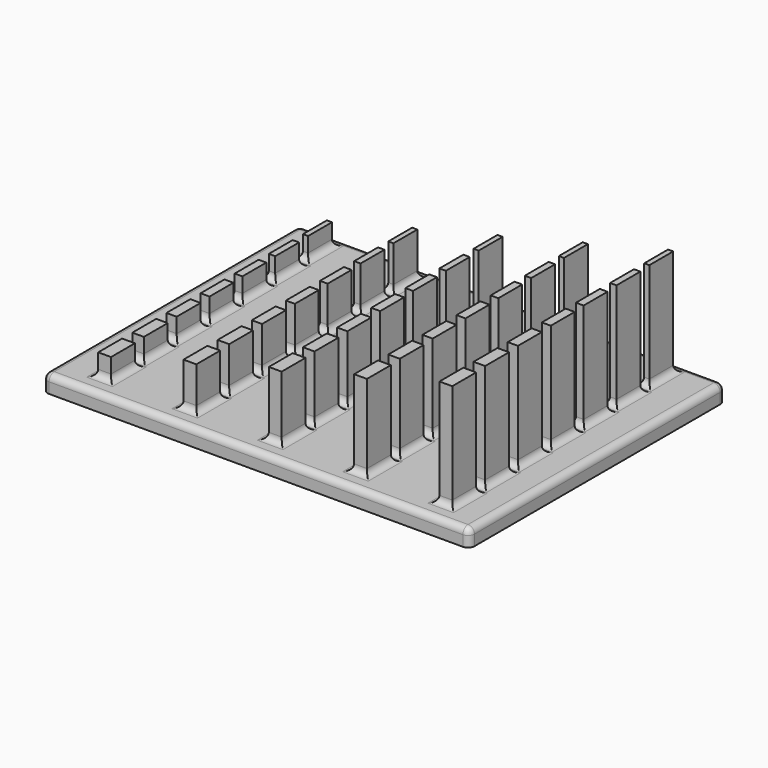
from build123d import *

# Parameters (mm, degrees)
F0_W          = 100
F0_H          = 75
F1_DEPTH      = 4
F2_W          = 2.4
F2_H          = 7
F2_W_2        = 3
F2_W_3        = 1.8
F2_W_4        = 1.2
F2_W_5        = 1.5
F2_W_6        = 2.7
F2_W_7        = 2.1
F3_DEPTH      = 5
F4_DEPTH      = 10
F5_DEPTH      = 15
F6_DEPTH      = 20
F7_DEPTH      = 25
F8_R          = 1.49999
F9_T1_DEPTH   = 7.75
F9_T4_ANGLE   = 90
F9_T6_ANGLE   = 90
F9_T8_ANGLE   = 90
F9_T10_ANGLE  = 90
F10_TEXT_SIZE = 9.9957049705
F11_DEPTH     = 0.5


# Not quite as in the source:
# - a fillet or chamfer that OpenCascade refuses, or shapes differently, is made with other operations: its cross-section is extruded or revolved along the edge and cut away or added
# - a fillet or chamfer is up to 0.001 mm smaller than in the source, because OpenCascade refuses the exact size
# - Text() gives the source's letters only with a copy of the font that has no kerning and outlines rounded to 1/6400 em; it was checked with that copy


with BuildPart() as f1:
    # F0 (on Top) → F1 (new body)
    with BuildSketch(Plane.XY):
        Rectangle(F0_W, F0_H)
    extrude(amount=F1_DEPTH)

    # F2 (on face) → F3 (join)
    with BuildSketch(Plane.XY.offset(4)):
        with Locations((-39.8, -9)):
            Rectangle(F2_W, F2_H)
        with Locations((-39.5, -29)):
            Rectangle(F2_W_2, F2_H)
        with Locations((-40.1, 11)):
            Rectangle(F2_W_3, F2_H)
        with Locations((-40.4, 31)):
            Rectangle(F2_W_4, F2_H)
        with Locations((-40.25, 21)):
            Rectangle(F2_W_5, F2_H)
        with Locations((-39.65, -19)):
            Rectangle(F2_W_6, F2_H)
        with Locations((-39.95, 1)):
            Rectangle(F2_W_7, F2_H)
    extrude(amount=F3_DEPTH)

    # F2 (on face) → F4 (join)
    with BuildSketch(Plane.XY.offset(4)):
        with Locations((-20.25, 21)):
            Rectangle(F2_W_5, F2_H)
        with Locations((-19.65, -19)):
            Rectangle(F2_W_6, F2_H)
        with Locations((-19.95, 1)):
            Rectangle(F2_W_7, F2_H)
        with Locations((-20.1, 11)):
            Rectangle(F2_W_3, F2_H)
        with Locations((-19.5, -29)):
            Rectangle(F2_W_2, F2_H)
        with Locations((-20.4, 31)):
            Rectangle(F2_W_4, F2_H)
        with Locations((-19.8, -9)):
            Rectangle(F2_W, F2_H)
    extrude(amount=F4_DEPTH)

    # F2 (on face) → F5 (join)
    with BuildSketch(Plane.XY.offset(4)):
        with Locations((-0.4, 31)):
            Rectangle(F2_W_4, F2_H)
        with Locations((-0.1, 11)):
            Rectangle(F2_W_3, F2_H)
        with Locations((0.2, -9)):
            Rectangle(F2_W, F2_H)
        with Locations((0.05, 1)):
            Rectangle(F2_W_7, F2_H)
        with Locations((-0.25, 21)):
            Rectangle(F2_W_5, F2_H)
        with Locations((0.35, -19)):
            Rectangle(F2_W_6, F2_H)
        with Locations((0.5, -29)):
            Rectangle(F2_W_2, F2_H)
    extrude(amount=F5_DEPTH)

    # F2 (on face) → F6 (join)
    with BuildSketch(Plane.XY.offset(4)):
        with Locations((19.6, 31)):
            Rectangle(F2_W_4, F2_H)
        with Locations((19.75, 21)):
            Rectangle(F2_W_5, F2_H)
        with Locations((20.2, -9)):
            Rectangle(F2_W, F2_H)
        with Locations((20.35, -19)):
            Rectangle(F2_W_6, F2_H)
        with Locations((20.5, -29)):
            Rectangle(F2_W_2, F2_H)
        with Locations((19.9, 11)):
            Rectangle(F2_W_3, F2_H)
        with Locations((20.05, 1)):
            Rectangle(F2_W_7, F2_H)
    extrude(amount=F6_DEPTH)

    # F2 (on face) → F7 (join)
    with BuildSketch(Plane.XY.offset(4)):
        with Locations((39.6, 31)):
            Rectangle(F2_W_4, F2_H)
        with Locations((39.75, 21)):
            Rectangle(F2_W_5, F2_H)
        with Locations((40.2, -9)):
            Rectangle(F2_W, F2_H)
        with Locations((40.05, 1)):
            Rectangle(F2_W_7, F2_H)
        with Locations((40.5, -29)):
            Rectangle(F2_W_2, F2_H)
        with Locations((39.9, 11)):
            Rectangle(F2_W_3, F2_H)
        with Locations((40.35, -19)):
            Rectangle(F2_W_6, F2_H)
    extrude(amount=F7_DEPTH)

    # F8 (radius 1.5 in the source; OpenCascade refuses exactly that, so slightly less here)
    f8_edges = [f1.edges().sort_by_distance(p)[0] for p in [
        (0, 37.5, 4),
        (50, 0, 4),
        (-50, 0, 4),
        (0, -37.5, 4),
        (-39.5, -25.5, 4),
        (-38, -29, 4),
        (-41, -29, 4),
        (-39.5, -32.5, 4),
        (-39.65, -15.5, 4),
        (-38.3, -19, 4),
        (-41, -19, 4),
        (-39.65, -22.5, 4),
        (-19.5, -25.5, 4),
        (-18, -29, 4),
        (-21, -29, 4),
        (-19.5, -32.5, 4),
        (-19.65, -15.5, 4),
        (-18.3, -19, 4),
        (-21, -19, 4),
        (-19.65, -22.5, 4),
        (0.35, -15.5, 4),
        (1.7, -19, 4),
        (-1, -19, 4),
        (0.35, -22.5, 4),
        (-39.8, -5.5, 4),
        (-38.6, -9, 4),
        (-41, -9, 4),
        (-39.8, -12.5, 4),
        (-19.8, -5.5, 4),
        (-18.6, -9, 4),
        (-21, -9, 4),
        (-19.8, -12.5, 4),
        (0.2, -5.5, 4),
        (1.4, -9, 4),
        (-1, -9, 4),
        (0.2, -12.5, 4),
        (0.5, -25.5, 4),
        (2, -29, 4),
        (-1, -29, 4),
        (0.5, -32.5, 4),
        (20.5, -25.5, 4),
        (22, -29, 4),
        (19, -29, 4),
        (20.5, -32.5, 4),
        (20.35, -15.5, 4),
        (21.7, -19, 4),
        (19, -19, 4),
        (20.35, -22.5, 4),
        (40.5, -25.5, 4),
        (39, -29, 4),
        (40.5, -32.5, 4),
        (42, -29, 4),
        (40.35, -15.5, 4),
        (39, -19, 4),
        (40.35, -22.5, 4),
        (41.7, -19, 4),
        (20.2, -5.5, 4),
        (21.4, -9, 4),
        (19, -9, 4),
        (20.2, -12.5, 4),
        (40.2, -5.5, 4),
        (39, -9, 4),
        (40.2, -12.5, 4),
        (41.4, -9, 4),
        (-39.95, 4.5, 4),
        (-38.9, 1, 4),
        (-41, 1, 4),
        (-39.95, -2.5, 4),
        (-40.1, 14.5, 4),
        (-39.2, 11, 4),
        (-41, 11, 4),
        (-40.1, 7.5, 4),
        (-18.9, 1, 4),
        (-19.95, -2.5, 4),
        (-19.95, 4.5, 4),
        (-21, 1, 4),
        (1.1, 1, 4),
        (0.05, -2.5, 4),
        (0.05, 4.5, 4),
        (-1, 1, 4),
        (-20.1, 14.5, 4),
        (-19.2, 11, 4),
        (-21, 11, 4),
        (-20.1, 7.5, 4),
        (-0.1, 14.5, 4),
        (0.8, 11, 4),
        (-1, 11, 4),
        (-0.1, 7.5, 4),
        (-40.25, 24.5, 4),
        (-39.5, 21, 4),
        (-41, 21, 4),
        (-40.25, 17.5, 4),
        (-40.4, 34.5, 4),
        (-39.8, 31, 4),
        (-41, 31, 4),
        (-40.4, 27.5, 4),
        (-20.4, 34.5, 4),
        (-19.8, 31, 4),
        (-21, 31, 4),
        (-20.4, 27.5, 4),
        (-19.5, 21, 4),
        (-20.25, 17.5, 4),
        (-20.25, 24.5, 4),
        (-21, 21, 4),
        (0.5, 21, 4),
        (-0.25, 17.5, 4),
        (-0.25, 24.5, 4),
        (-1, 21, 4),
        (-0.4, 34.5, 4),
        (0.2, 31, 4),
        (-1, 31, 4),
        (-0.4, 27.5, 4),
        (21.1, 1, 4),
        (20.05, -2.5, 4),
        (20.05, 4.5, 4),
        (19, 1, 4),
        (19.9, 14.5, 4),
        (20.8, 11, 4),
        (19, 11, 4),
        (19.9, 7.5, 4),
        (41.1, 1, 4),
        (40.05, 4.5, 4),
        (39, 1, 4),
        (40.05, -2.5, 4),
        (39.9, 14.5, 4),
        (39, 11, 4),
        (39.9, 7.5, 4),
        (40.8, 11, 4),
        (20.5, 21, 4),
        (19.75, 17.5, 4),
        (19.75, 24.5, 4),
        (19, 21, 4),
        (19.6, 34.5, 4),
        (20.2, 31, 4),
        (19, 31, 4),
        (19.6, 27.5, 4),
        (40.5, 21, 4),
        (39.75, 24.5, 4),
        (39, 21, 4),
        (39.75, 17.5, 4),
        (39.6, 34.5, 4),
        (39, 31, 4),
        (39.6, 27.5, 4),
        (40.2, 31, 4),
    ]]
    fillet(f8_edges, radius=F8_R)

    # F9: fillet of radius 1.5 on 4 edges, made by hand

    # F9_s2 → F9_t1 (cut)
    with BuildSketch(Plane.XY.offset(-3.75)):
        with BuildLine():
            ThreePointArc((-48.5, 37.5), (-49.5606601718, 37.0606601718), (-50, 36))
            Line((-50, 36), (-50, 37.5))
            Line((-50, 37.5), (-48.5, 37.5))
        make_face()
        with BuildLine():
            ThreePointArc((48.5, 37.5), (49.5606601718, 37.0606601718), (50, 36))
            Line((50, 36), (50, 37.5))
            Line((50, 37.5), (48.5, 37.5))
        make_face()
        with BuildLine():
            ThreePointArc((50, -36), (49.5606601718, -37.0606601718), (48.5, -37.5))
            Line((48.5, -37.5), (50, -37.5))
            Line((50, -37.5), (50, -36))
        make_face()
        with BuildLine():
            ThreePointArc((-50, -36), (-49.5606601718, -37.0606601718), (-48.5, -37.5))
            Line((-48.5, -37.5), (-50, -37.5))
            Line((-50, -37.5), (-50, -36))
        make_face()
    extrude(amount=F9_T1_DEPTH, mode=Mode.SUBTRACT)

    # F9_s3 → F9_t4 (revolve, cut)
    with BuildSketch(Plane.XZ.offset(36)):
        with BuildLine():
            ThreePointArc((-48.50001, 4), (-49.5606631007, 3.5606631007), (-50, 2.50001))
            Line((-50, 2.50001), (-50, 4))
            Line((-50, 4), (-48.50001, 4))
        make_face()
    revolve(axis=Axis((-48.5, -36, 4), (0, 0, 1)), revolution_arc=F9_T4_ANGLE, mode=Mode.SUBTRACT)

    # F9_s5 → F9_t6 (revolve, cut)
    with BuildSketch(Plane.YZ.offset(48.5)):
        with BuildLine():
            ThreePointArc((-36.00001, 4), (-37.0606631007, 3.5606631007), (-37.5, 2.50001))
            Line((-37.5, 2.50001), (-37.5, 4))
            Line((-37.5, 4), (-36.00001, 4))
        make_face()
    revolve(axis=Axis((48.5, -36, 4), (0, 0, 1)), revolution_arc=F9_T6_ANGLE, mode=Mode.SUBTRACT)

    # F9_s7 → F9_t8 (revolve, cut)
    with BuildSketch(Plane.XZ.offset(-36)):
        with BuildLine():
            ThreePointArc((48.50001, 4), (49.5606631007, 3.5606631007), (50, 2.50001))
            Line((50, 2.50001), (50, 4))
            Line((50, 4), (48.50001, 4))
        make_face()
    revolve(axis=Axis((48.5, 36, 4), (0, 0, 1)), revolution_arc=F9_T8_ANGLE, mode=Mode.SUBTRACT)

    # F9_s9 → F9_t10 (revolve, cut)
    with BuildSketch(Plane.YZ.offset(-48.5)):
        with BuildLine():
            ThreePointArc((36.00001, 4), (37.0606631007, 3.5606631007), (37.5, 2.50001))
            Line((37.5, 2.50001), (37.5, 4))
            Line((37.5, 4), (36.00001, 4))
        make_face()
    revolve(axis=Axis((-48.5, 36, 4), (0, 0, 1)), revolution_arc=F9_T10_ANGLE, mode=Mode.SUBTRACT)

    # F10 (on face) → F11 (cut)
    with BuildSketch(Plane(origin=(0, 0, 0), x_dir=(1, 0, 0), z_dir=(0, 0, -1))):
        with Locations((-40, -3.0863287755)):
            Text('SNAP TEST 001-A', F10_TEXT_SIZE, font='Open Sans', text_align=(TextAlign.LEFT, TextAlign.BOTTOM))
    extrude(amount=-F11_DEPTH, mode=Mode.SUBTRACT)


solid = f1.part
